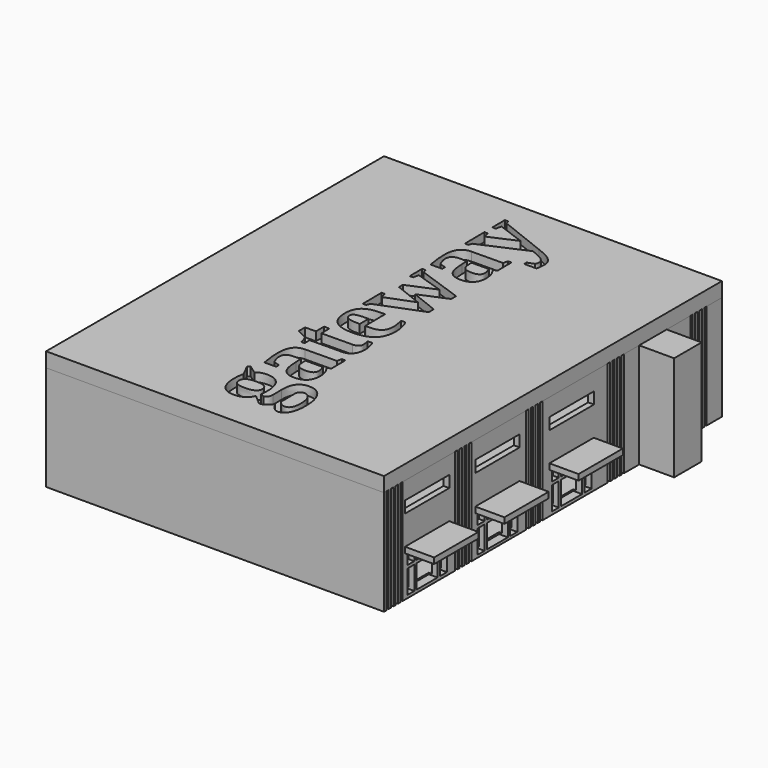
from build123d import *

# Parameters (mm, degrees)
F0_W         = 116
F0_H         = 145
F1_DEPTH     = 36
F2_T         = -3
F3_W         = 116
F3_H         = 145
F4_DEPTH     = 5
F5_W         = 5
F5_H         = 5
F6_DEPTH     = 10
F7_W         = 5
F7_H         = 5
F8_DEPTH     = 10
F9_TEXT_SIZE = 36.1193359702
F10_DEPTH    = 3
F11_W        = 1
F11_H        = 36
F12_DEPTH    = 1
F13_W        = 3
F13_H        = 3
F13_W_2      = 9
F13_H_2      = 8
F13_H_3      = 8.0094143525
F13_W_3      = 3.0275415629
F14_DEPTH    = 3
F13_W_4      = 19
F13_H_4      = 2
F15_DEPTH    = 10
F13_W_5      = 11.7830485106
F13_H_5      = 36
F16_DEPTH    = 12
F17_W        = 1
F17_H        = 36
F18_DEPTH    = 1
F19_DEPTH    = 1
F20_W        = 19
F20_H        = 4
F21_DEPTH    = 5
F23_DEPTH    = 1.5
F24_W        = 110
F24_H        = 34.5
F25_DEPTH    = 1.5
F26_W        = 140.5
F26_H        = 34.5
F27_DEPTH    = 1.5
F28_W        = 111.5
F28_H        = 34.5
F29_DEPTH    = 1.5
F30_W        = 3
F30_H        = 3
F30_W_2      = 9
F30_W_3      = 19
F30_H_2      = 4
F31_DEPTH    = 1


# Not quite as in the source:
# - Text() gives the source's letters only with a copy of the font that has no kerning and outlines rounded to 1/6400 em; it was checked with that copy


with BuildPart() as f1:
    # F0 (on Top) → F1 (new body)
    with BuildSketch(Plane.XY):
        with Locations((-58, 72.5)):
            Rectangle(F0_W, F0_H)
    extrude(amount=F1_DEPTH)

    # F2
    f2_openings = [f1.faces().sort_by_distance(p)[0] for p in [
        (-58, 72.5, 36),
    ]]
    offset(amount=F2_T, openings=f2_openings)

    # F11 (on face) → F12 (cut)
    with BuildSketch(Plane.YZ):
        with Locations((1.5, 18)):
            Rectangle(F11_W, F11_H)
        with Locations((3.5, 18)):
            Rectangle(F11_W, F11_H)
        with Locations((5.4932315014, 18)):
            Rectangle(F11_W, F11_H)
        with Locations((7.4932315014, 18)):
            Rectangle(F11_W, F11_H)
    extrude(amount=-F12_DEPTH, mode=Mode.SUBTRACT)

    # F13 (on face) → F14 (cut)
    with BuildSketch(Plane.YZ):
        with Locations((11.5, 11.5)):
            Rectangle(F13_W, F13_H)
        with Locations((18.5, 11.5)):
            Rectangle(F13_W_2, F13_H)
        with Locations((25.5, 11.5)):
            Rectangle(F13_W, F13_H)
        with Locations((25.5, 5)):
            Rectangle(F13_W, F13_H_2)
        with Locations((18.5, 5.0047071762)):
            Rectangle(F13_W_2, F13_H_3)
        with Locations((11.5, 5)):
            Rectangle(F13_W, F13_H_2)
        with Locations((41.6610901324, 11.3798414679)):
            Rectangle(F13_W, F13_H)
        with Locations((48.6610901324, 11.3798414679)):
            Rectangle(F13_W_2, F13_H)
        with Locations((55.6610901324, 11.3798414679)):
            Rectangle(F13_W, F13_H)
        with Locations((55.6748609138, 4.8798414679)):
            Rectangle(F13_W_3, F13_H_2)
        with Locations((48.6610901324, 4.8845486441)):
            Rectangle(F13_W_2, F13_H_3)
        with Locations((41.6610901324, 4.8798414679)):
            Rectangle(F13_W, F13_H_2)
        with Locations((73.4838088123, 11.5129751941)):
            Rectangle(F13_W, F13_H)
        with Locations((80.4838088123, 11.5129751941)):
            Rectangle(F13_W_2, F13_H)
        with Locations((87.4838088123, 11.5129751941)):
            Rectangle(F13_W, F13_H)
        with Locations((87.4975795937, 5.0129751941)):
            Rectangle(F13_W_3, F13_H_2)
        with Locations((80.4838088123, 5.0176823703)):
            Rectangle(F13_W_2, F13_H_3)
        with Locations((73.4838088123, 5.0129751941)):
            Rectangle(F13_W, F13_H_2)
    extrude(amount=-F14_DEPTH, mode=Mode.SUBTRACT)

    # F13 (on face) → F15 (join)
    with BuildSketch(Plane.YZ):
        with Locations((80.4838088123, 15.0129751941)):
            Rectangle(F13_W_4, F13_H_4)
        with Locations((48.6610901324, 14.8798414679)):
            Rectangle(F13_W_4, F13_H_4)
        with Locations((18.5, 15)):
            Rectangle(F13_W_4, F13_H_4)
    extrude(amount=F15_DEPTH)

    # F13 (on face) → F16 (join)
    with BuildSketch(Plane.YZ):
        with Locations((115.3852641582, 18)):
            Rectangle(F13_W_5, F13_H_5)
    extrude(amount=F16_DEPTH)

    # F17 (on face) → F18 (cut)
    with BuildSketch(Plane.YZ):
        with Locations((31, 18)):
            Rectangle(F17_W, F17_H)
        with Locations((33, 18)):
            Rectangle(F17_W, F17_H)
        with Locations((35, 18)):
            Rectangle(F17_W, F17_H)
        with Locations((37, 18)):
            Rectangle(F17_W, F17_H)
        with Locations((61.4838088123, 18)):
            Rectangle(F17_W, F17_H)
        with Locations((63.4838088123, 18)):
            Rectangle(F17_W, F17_H)
        with Locations((65.4838088123, 18)):
            Rectangle(F17_W, F17_H)
        with Locations((67.4838088123, 18)):
            Rectangle(F17_W, F17_H)
    extrude(amount=-F18_DEPTH, mode=Mode.SUBTRACT)

    # F17 (on face) → F19 (cut)
    with BuildSketch(Plane.YZ):
        with Locations((96.4838107228, 18)):
            Rectangle(F17_W, F17_H)
        with Locations((98.4838107228, 18)):
            Rectangle(F17_W, F17_H)
        with Locations((100.4838107228, 18)):
            Rectangle(F17_W, F17_H)
        with Locations((102.4838107228, 18)):
            Rectangle(F17_W, F17_H)
        with Locations((131.956553936, 18)):
            Rectangle(F17_W, F17_H)
        with Locations((133.956553936, 18)):
            Rectangle(F17_W, F17_H)
        with Locations((135.956553936, 18)):
            Rectangle(F17_W, F17_H)
        with Locations((137.956553936, 18)):
            Rectangle(F17_W, F17_H)
    extrude(amount=-F19_DEPTH, mode=Mode.SUBTRACT)

    # F20 (on face) → F21 (cut)
    with BuildSketch(Plane.YZ):
        with Locations((18.5, 28)):
            Rectangle(F20_W, F20_H)
        with Locations((48.7255485058, 28)):
            Rectangle(F20_W, F20_H)
        with Locations((80.6086243391, 28)):
            Rectangle(F20_W, F20_H)
    extrude(amount=-F21_DEPTH, mode=Mode.SUBTRACT)

    # F22 (on face) → F23 (cut)
    with BuildSketch(Plane.XY.offset(3)):
        Polygon((-113, 142), (-113, 3), (-3, 3), (-3, 10), (-3, 13), (-3, 14), (-3, 23), (-3, 24), (-3, 27), (-3, 40.1610901324), (-3, 43.1610901324), (-3, 44.1610901324), (-3, 53.1610901324), (-3, 54.1610901324), (-3, 57.1886316953), (-3, 71.9838088123), (-3, 74.9838088123), (-3, 75.9838088123), (-3, 84.9838088123), (-3, 85.9838088123), (-3, 89.0113503752), (-3, 142), align=None)
    extrude(amount=-F23_DEPTH, mode=Mode.SUBTRACT)

    # F24 (on face) → F25 (cut)
    with BuildSketch(Plane.XZ.offset(-142)):
        with Locations((-58, 18.75)):
            Rectangle(F24_W, F24_H)
    extrude(amount=-F25_DEPTH, mode=Mode.SUBTRACT)

    # F26 (on face) → F27 (cut)
    with BuildSketch(Plane.YZ.offset(-113)):
        with Locations((73.25, 18.75)):
            Rectangle(F26_W, F26_H)
    extrude(amount=-F27_DEPTH, mode=Mode.SUBTRACT)

    # F28 (on face) → F29 (cut)
    with BuildSketch(Plane(origin=(0, 3, 0), x_dir=(-1, 0, 0), z_dir=(0, 1, 0))):
        with Locations((58.75, 18.75)):
            Rectangle(F28_W, F28_H)
    extrude(amount=-F29_DEPTH, mode=Mode.SUBTRACT)

    # F30 (on face) → F31 (cut)
    with BuildSketch(Plane(origin=(-3, 0, 0), x_dir=(0, -1, 0), z_dir=(-1, 0, 0))):
        Polygon((-10, 1.5), (-1.5, 1.5), (-1.5, 36), (-143.5, 36), (-143.5, 1.5), (-89.0113503752, 1.5), (-89.0113503752, 9.0129751941), (-85.9838088123, 9.0129751941), (-85.9838088123, 1.5), (-84.9838088123, 1.5), (-84.9838088123, 9.0223895466), (-75.9838088123, 9.0223895466), (-75.9838088123, 1.5), (-74.9838088123, 1.5), (-74.9838088123, 9.0129751941), (-71.9838088123, 9.0129751941), (-71.9838088123, 1.5), (-57.1886316953, 1.5), (-57.1886316953, 8.8798414679), (-54.1610901324, 8.8798414679), (-54.1610901324, 1.5), (-53.1610901324, 1.5), (-53.1610901324, 8.8892558204), (-44.1610901324, 8.8892558204), (-44.1610901324, 1.5), (-43.1610901324, 1.5), (-43.1610901324, 8.8798414679), (-40.1610901324, 8.8798414679), (-40.1610901324, 1.5), (-27, 1.5), (-27, 9), (-24, 9), (-24, 1.5), (-23, 1.5), (-23, 9.0094143525), (-14, 9.0094143525), (-14, 1.5), (-13, 1.5), (-13, 9), (-10, 9), align=None)
        with Locations((-87.4838088123, 11.5129751941)):
            Rectangle(F30_W, F30_H, mode=Mode.SUBTRACT)
        with Locations((-80.4838088123, 11.5129751941)):
            Rectangle(F30_W_2, F30_H, mode=Mode.SUBTRACT)
        with Locations((-73.4838088123, 11.5129751941)):
            Rectangle(F30_W, F30_H, mode=Mode.SUBTRACT)
        with Locations((-55.6610901324, 11.3798414679)):
            Rectangle(F30_W, F30_H, mode=Mode.SUBTRACT)
        with Locations((-48.6610901324, 11.3798414679)):
            Rectangle(F30_W_2, F30_H, mode=Mode.SUBTRACT)
        with Locations((-41.6610901324, 11.3798414679)):
            Rectangle(F30_W, F30_H, mode=Mode.SUBTRACT)
        with Locations((-25.5, 11.5)):
            Rectangle(F30_W, F30_H, mode=Mode.SUBTRACT)
        with Locations((-18.5, 11.5)):
            Rectangle(F30_W_2, F30_H, mode=Mode.SUBTRACT)
        with Locations((-11.5, 11.5)):
            Rectangle(F30_W, F30_H, mode=Mode.SUBTRACT)
        with Locations((-80.6086243391, 28)):
            Rectangle(F30_W_3, F30_H_2, mode=Mode.SUBTRACT)
        with Locations((-48.7255485058, 28)):
            Rectangle(F30_W_3, F30_H_2, mode=Mode.SUBTRACT)
        with Locations((-18.5, 28)):
            Rectangle(F30_W_3, F30_H_2, mode=Mode.SUBTRACT)
    extrude(amount=-F31_DEPTH, mode=Mode.SUBTRACT)


with BuildPart() as f4:
    # F3 (on face) → F4 (new body)
    with BuildSketch(Plane.XY.offset(36)):
        with Locations((-58, 72.5)):
            Rectangle(F3_W, F3_H)
    extrude(amount=F4_DEPTH)

    # F5 (on face) → F6 (join)
    with BuildSketch(Plane.XY.offset(41)):
        with Locations((-110.4, 5.6)):
            Rectangle(F5_W, F5_H)
    extrude(amount=-F6_DEPTH)

    # F7 (on face) → F8 (join)
    with BuildSketch(Plane.XY.offset(41)):
        with Locations((-5.6, 139.4)):
            Rectangle(F7_W, F7_H)
    extrude(amount=-F8_DEPTH)

    # F9 (on face) → F10 (cut)
    with BuildSketch(Plane.XY.offset(41)):
        with Locations(Location((-49.7102085501, 10.4342792183), (0, 0, 90.5750930101))):
            Text('gateway', F9_TEXT_SIZE, font='Tinos', font_style=FontStyle.BOLD, text_align=(TextAlign.LEFT, TextAlign.BOTTOM))
    extrude(amount=-F10_DEPTH, mode=Mode.SUBTRACT)


solid = Compound([f1.part, f4.part])
